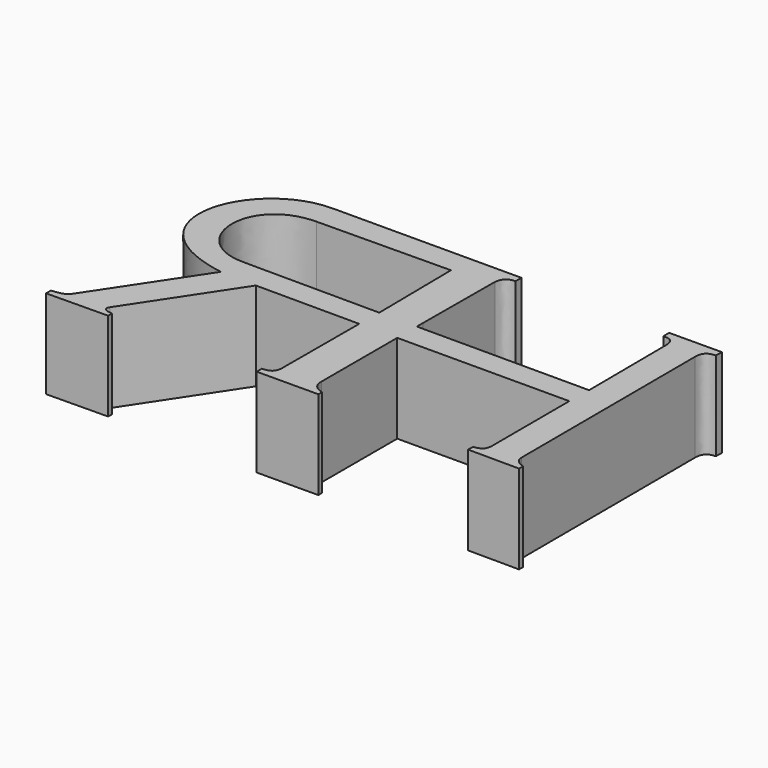
from build123d import *

# Parameters (mm, degrees)
F1_DEPTH = 3


# Not quite as in the source:
# - ends of sketch curves that miss each other by under 0.0002 mm in the source are joined


with BuildPart() as f1:
    # F0 (on Top) → F1 (new body)
    with BuildSketch(Plane.XY):
        with BuildLine():
            Line((1.1892447866, 4.276448), (-5.1239697534, 4.2621811105))
            add(Edge.make_bspline(
                [(-5.1239697534, 4.2621811105), (-7.7808246997, 4.2757478261), (-9.2426975653, 0.2504639081), (-5.1792210147, -0.4118392886)],
                knots=[0, 0, 0, 0, 1, 1, 1, 1], degree=3))
            Line((-5.1792210147, -0.4118392886), (-7.4358199708, -3.8138012247))
            add(Edge.make_bspline(
                [(-7.4358199708, -3.8138012247), (-7.5115597505, -3.9074856806), (-7.537762832, -4.0076449282), (-8.0121770072, -4.0492147307)],
                knots=[0, 0, 0, 0, 1, 1, 1, 1], degree=3))
            Line((-8.0121770072, -4.0492147307), (-8.0121770072, -4.2521576986))
            Line((-8.0121770072, -4.2521576986), (-5.9340439579, -4.2278042412))
            Line((-5.9340439579, -4.2278042412), (-5.9340439579, -4.0654502213))
            add(Edge.make_bspline(
                [(-5.9340439579, -4.0654502213), (-6.0599730098, -4.054522155), (-6.1436827864, -4.0293012572), (-6.1809375378, -4.0026613543)],
                knots=[0, 0, 0, 0, 1, 1, 1, 1], degree=3))
            add(Edge.make_bspline(
                [(-6.1809375378, -4.0026613543), (-6.2530914835, -3.9629456061), (-6.2541383485, -3.9018136478), (-6.2019284451, -3.8219191915)],
                knots=[0, 0, 0, 0, 1, 1, 1, 1], degree=3))
            Line((-6.2019284451, -3.8219191915), (-3.9695588998, -0.4449526542))
            Line((-3.9695588998, -0.4449526542), (-0.4708268475, -0.453070178))
            Line((-0.4708268475, -0.453070178), (-0.4789443713, -3.7001536766))
            add(Edge.make_bspline(
                [(-0.4789443713, -3.7001536766), (-0.4894063767, -3.8582816931), (-0.511182765, -4.0522109002), (-0.8767118972, -4.0573326976)],
                knots=[0, 0, 0, 0, 1, 1, 1, 1], degree=3))
            Line((-0.8767118972, -4.0573326976), (-0.8767118972, -4.276510713))
            Line((-0.8767118972, -4.276510713), (1.2014211521, -4.2683931892))
            Line((1.2014211521, -4.2683931892), (1.2009267376, -4.1117789848))
            add(Edge.make_bspline(
                [(1.2009267376, -4.1117789848), (0.9540548658, -4.0521630537), (0.8074211, -3.9109443668), (0.8117693779, -3.643329238)],
                knots=[0, 0, 0, 0, 1, 1, 1, 1], degree=3))
            Line((0.8117693779, -3.643329238), (0.8117693779, -0.4504044473))
            Line((0.8117693779, -0.4504044473), (6.6162368382, -0.4383405203))
            Line((6.6162368382, -0.4383405203), (6.623033018, -3.7082712004))
            add(Edge.make_bspline(
                [(6.623033018, -3.7082712004), (6.6159065383, -3.8428631383), (6.6131664366, -4.0230470912), (6.2638249484, -4.0654502213)],
                knots=[0, 0, 0, 0, 1, 1, 1, 1], degree=3))
            Line((6.2638249484, -4.0654502213), (6.2587514407, -4.2683931892))
            Line((6.2587514407, -4.2683931892), (7.9878229928, -4.276510713))
            Line((7.9878229928, -4.276510713), (7.9878229928, -4.1060387263))
            add(Edge.make_bspline(
                [(7.9878229928, -4.1060387263), (7.7941463093, -4.0440123031), (7.6495123525, -3.9453779431), (7.6468790194, -3.7407417386)],
                knots=[0, 0, 0, 0, 1, 1, 1, 1], degree=3))
            Line((7.6468790194, -3.7407417386), (7.6225260051, 3.6139009438))
            add(Edge.make_bspline(
                [(7.6225260051, 3.6139009438), (7.6218814055, 3.8627278793), (7.729467946, 4.0122785134), (8.0040584834, 4.0164664167)],
                knots=[0, 0, 0, 0, 1, 1, 1, 1], degree=3))
            Line((8.0040584834, 4.0164664167), (8.0121760072, 4.2633179094))
            Line((8.0121760072, 4.2633179094), (6.2343979833, 4.2551999426))
            Line((6.2343979833, 4.2551999426), (6.2363273516, 4.008799005))
            add(Edge.make_bspline(
                [(6.2363273516, 4.008799005), (6.3452247993, 4.0058905543), (6.6002611554, 4.0485187405), (6.6097418632, 3.6759729985)],
                knots=[0, 0, 0, 0, 1, 1, 1, 1], degree=3))
            Line((6.6097418632, 3.6759729985), (6.6321672813, 0.5291723511))
            Line((6.6321672813, 0.5291723511), (6.6332519216, 0.3769724351))
            Line((6.6332519216, 0.3769724351), (0.8123838086, 0.3769724351))
            Line((0.8123838086, 0.3769724351), (0.8123838086, 0.6393006265))
            Line((0.8123838086, 0.6393006265), (0.8280061975, 3.6544898918))
            add(Edge.make_bspline(
                [(0.8280061975, 3.6544898918), (0.8551715265, 3.8458646241), (0.9207173302, 4.0128832408), (1.2257741664, 4.0279044033)],
                knots=[0, 0, 0, 0, 1, 1, 1, 1], degree=3))
            Line((1.2257741664, 4.0279044033), (1.2328771659, 4.2765093839))
            Line((1.2328771659, 4.2765093839), (1.2099382837, 4.2765100827))
            Line((1.2099382837, 4.2765100827), (1.1892447866, 4.276448))
        make_face()
        with BuildLine():
            Line((-0.456683315, 0.3769724351), (-5.024860472, 0.3920733419))
            add(Edge.make_bspline(
                [(-5.024860472, 0.3920733419), (-7.1084099294, 0.3583060733), (-7.3152098618, 3.3560575894), (-5.0022086687, 3.4048052624)],
                knots=[0, 0, 0, 0, 1, 1, 1, 1], degree=3))
            Line((-5.0022086687, 3.4048052624), (-0.4944369111, 3.450109312))
            Line((-0.4944369111, 3.450109312), (-0.456683315, 0.3769724351))
        make_face(mode=Mode.SUBTRACT)
    extrude(amount=F1_DEPTH)


solid = f1.part
